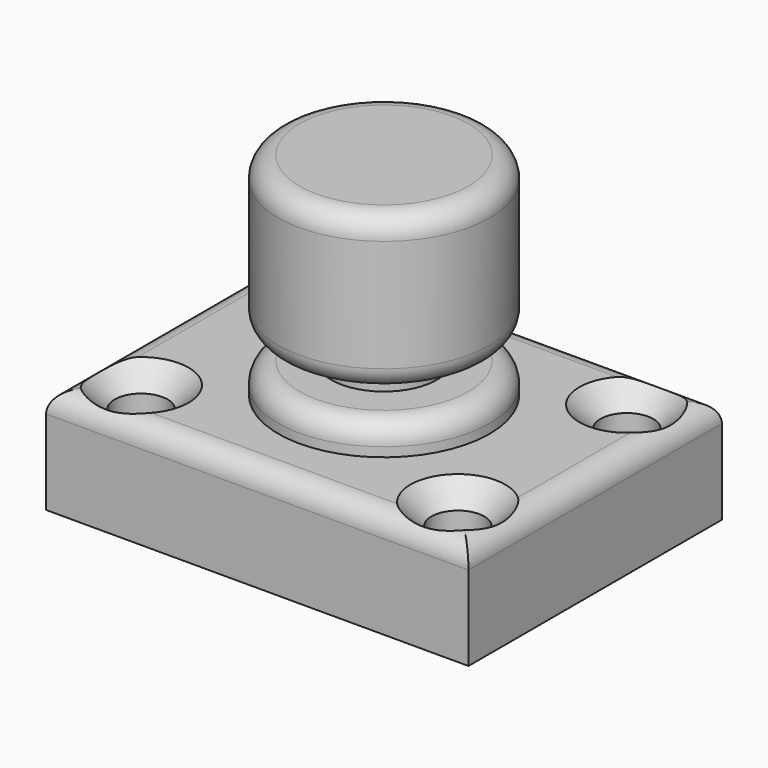
from build123d import *

# Parameters (mm, degrees)
F0_W     = 101.6
F0_H     = 76.2
F1_DEPTH = 25.4
F2_R     = 6.35
F3_DEPTH = 25.4
F4_R     = 25.4
F5_DEPTH = 50.8
F6_W     = 61.2722363651
F6_H     = 6.35
F8_R     = 5.08


# Not quite as in the source:
# - a fillet or chamfer that OpenCascade refuses, or shapes differently, is made with other operations: its cross-section is extruded or revolved along the edge and cut away or added


with BuildPart() as f1:
    # F0 (on Top) → F1 (new body)
    with BuildSketch(Plane.XY):
        Rectangle(F0_W, F0_H)
    extrude(amount=F1_DEPTH)

    # F2 (on face) → F3 (cut, through all)
    with BuildSketch(Plane.XY.offset(25.4)):
        with Locations((-38.1, 25.4)):
            Circle(F2_R)
        with Locations((38.1, 25.4)):
            Circle(F2_R)
        with Locations((38.1, -25.4)):
            Circle(F2_R)
        with Locations((-38.1, -25.4)):
            Circle(F2_R)
    extrude(amount=-F3_DEPTH, mode=Mode.SUBTRACT)

    # F4 (on face) → F5 (join)
    with BuildSketch(Plane.XY.offset(25.4)):
        Circle(F4_R)
    extrude(amount=F5_DEPTH)

    # F6 (on Front) → F7 (revolve, cut)
    with BuildSketch(Plane.XZ):
        with Locations((-43.3361181825, 35.8842967927)):
            Rectangle(F6_W, F6_H)
    revolve(axis=Axis((0, 0, 28.4035503864), (0, 0, 1)), mode=Mode.SUBTRACT)

    # F8
    f8_edges = [f1.edges().sort_by_distance(p)[0] for p in [
        (0, -38.1, 25.4),
        (-25.4, 0, 32.709297),
        (-25.4, 0, 39.059297),
        (-25.4, 0, 76.2),
        (50.8, 0, 25.4),
        (0, 38.1, 25.4),
        (-50.8, 0, 25.4),
    ]]
    fillet(f8_edges, radius=F8_R)

    # F9: chamfer of 5.08 on 12 edges, made by hand

    # F9_s1 → F9_t2 (revolve, cut)
    with BuildSketch(Plane.XZ.offset(25.4)):
        Polygon((-26.67, 25.4), (-31.75, 20.32), (-31.75, 25.4), align=None)
    revolve(axis=Axis((-38.1, -25.4, 25.4), (0, 0, 1)), mode=Mode.SUBTRACT)

    # F9_s3 → F9_t4 (revolve, cut)
    with BuildSketch(Plane.XZ.offset(25.4)):
        Polygon((-26.67, 0), (-31.75, 5.08), (-31.75, 0), align=None)
    revolve(axis=Axis((-38.1, -25.4, 0), (0, 0, 1)), mode=Mode.SUBTRACT)

    # F9_s5 → F9_t6 (revolve, cut)
    with BuildSketch(Plane.XZ.offset(-25.4)):
        Polygon((-26.67, 25.4), (-31.75, 20.32), (-31.75, 25.4), align=None)
    revolve(axis=Axis((-38.1, 25.4, 25.4), (0, 0, 1)), mode=Mode.SUBTRACT)

    # F9_s7 → F9_t8 (revolve, cut)
    with BuildSketch(Plane.XZ.offset(-25.4)):
        Polygon((-26.67, 0), (-31.75, 5.08), (-31.75, 0), align=None)
    revolve(axis=Axis((-38.1, 25.4, 0), (0, 0, 1)), mode=Mode.SUBTRACT)

    # F9_s9 → F9_t10 (revolve, cut)
    with BuildSketch(Plane.XZ.offset(-25.4)):
        Polygon((49.53, 25.4), (44.45, 20.32), (44.45, 25.4), align=None)
    revolve(axis=Axis((38.1, 25.4, 25.4), (0, 0, 1)), mode=Mode.SUBTRACT)

    # F9_s11 → F9_t12 (revolve, cut)
    with BuildSketch(Plane.XZ.offset(-25.4)):
        Polygon((49.53, 0), (44.45, 5.08), (44.45, 0), align=None)
    revolve(axis=Axis((38.1, 25.4, 0), (0, 0, 1)), mode=Mode.SUBTRACT)

    # F9_s13 → F9_t14 (revolve, cut)
    with BuildSketch(Plane.XZ.offset(25.4)):
        Polygon((49.53, 25.4), (44.45, 20.32), (44.45, 25.4), align=None)
    revolve(axis=Axis((38.1, -25.4, 25.4), (0, 0, 1)), mode=Mode.SUBTRACT)

    # F9_s15 → F9_t16 (revolve, cut)
    with BuildSketch(Plane.XZ.offset(25.4)):
        Polygon((49.53, 0), (44.45, 5.08), (44.45, 0), align=None)
    revolve(axis=Axis((38.1, -25.4, 0), (0, 0, 1)), mode=Mode.SUBTRACT)


solid = f1.part
